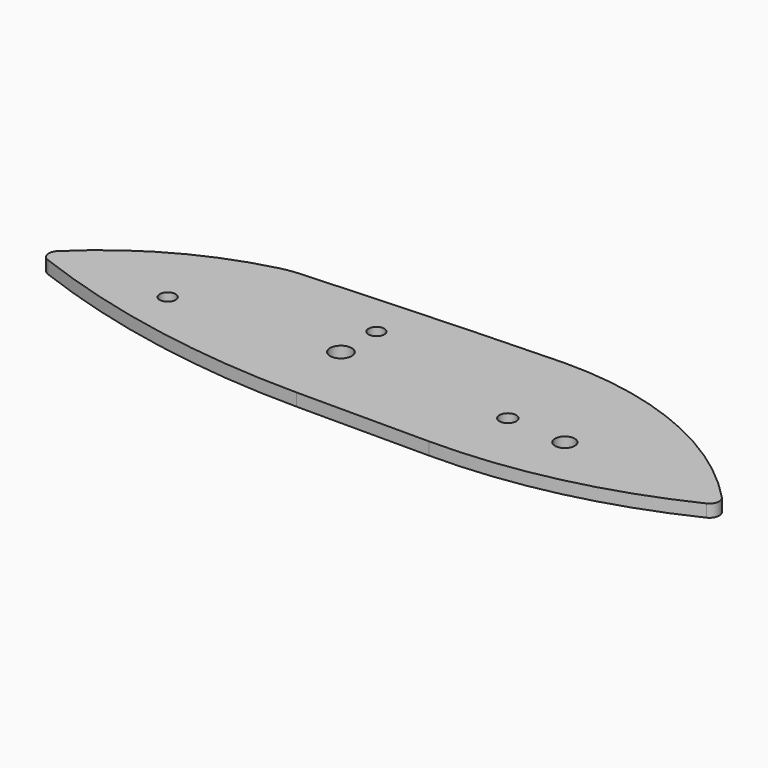
from build123d import *

# Parameters (mm, degrees)
F0_R     = 4.025
F0_R_2   = 5.5
F0_R_3   = 4.25
F0_R_4   = 5
F0_R_5   = 4
F1_DEPTH = 6.35


# Not quite as in the source:
# - a length typed as a fraction of an inch, garbled in the dataset ("3 / 203.2 mm" for 3/8 in), is restored


with BuildPart() as f1:
    # F0 (on Top) → F1 (new body)
    with BuildSketch(Plane.XY):
        with BuildLine():
            ThreePointArc((7.0672459204, -2.7674484319), (79.7907725168, -23.1351403858), (155, -30))
            Line((155, -30), (222, -30))
            ThreePointArc((222, -30), (283.0205715955, -23.1551675229), (341.0080980578, -2.9608944665))
            ThreePointArc((341.0080980578, -2.9608944665), (343.7637603339, 0.6365005197), (342.4812933157, 4.982786706))
            ThreePointArc((342.4812933157, 4.982786706), (287.5845162749, 43.1113755357), (222, 56))
            ThreePointArc((222, 56), (157.0912257731, 53.5938902672), (92.2239851956, 50.2503239761))
            ThreePointArc((92.2239851956, 50.2503239761), (87.6396110054, 49.7679486163), (83.1191443173, 48.8654223701))
            ThreePointArc((83.1191443173, 48.8654223701), (41.3356630681, 32.3684999851), (5.3506191001, 5.478271944))
            ThreePointArc((5.3506191001, 5.478271944), (3.9527325419, 0.8857070849), (7.0672459204, -2.7674484319))
        make_face()
        with Locations((64, 2)):
            Circle(F0_R, mode=Mode.SUBTRACT)
        with Locations((147, 8)):
            Circle(F0_R_2, mode=Mode.SUBTRACT)
        with Locations((234, 5)):
            Circle(F0_R_3, mode=Mode.SUBTRACT)
        with Locations((264.5, 3)):
            Circle(F0_R_4, mode=Mode.SUBTRACT)
        with Locations((147, 30.5)):
            Circle(F0_R_5, mode=Mode.SUBTRACT)
    extrude(amount=F1_DEPTH)


solid = f1.part
